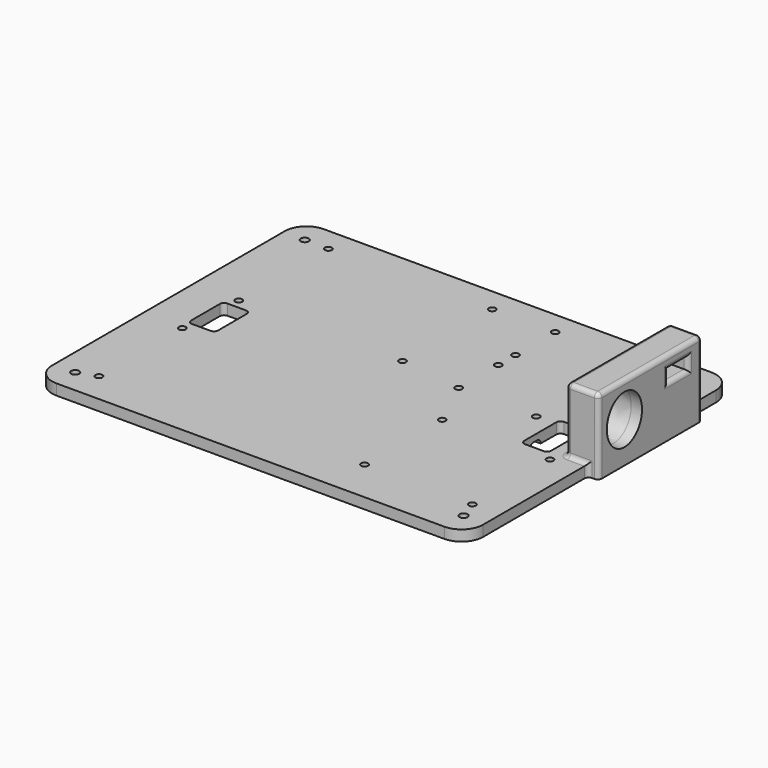
from build123d import *

# Parameters (mm, degrees)
F1_DEPTH  = 5
F2_R      = 1.85
F3_DEPTH  = 5
F2_R_2    = 2.595
F4_DEPTH  = 1.3
F5_DEPTH  = 2.17
F6_R      = 1.6
F7_DEPTH  = 3
F8_DEPTH  = 5
F9_W      = 12.5
F9_H      = 20.5508316867
F9_H_2    = 22.5
F10_DEPTH = 5
F9_W_2    = 10
F9_H_3    = 60
F9_W_3    = 5
F11_DEPTH = 30
F12_DEPTH = 5
F14_DEPTH = 10
F15_DEPTH = 5
F13_W     = 11.7
F13_H     = 5.3
F16_DEPTH = 10
F17_DEPTH = 5
F18_R     = 2
F19_R     = 2
F20_R     = 2


with BuildPart() as f1:
    # F0 (on Top) → F1 (new body)
    with BuildSketch(Plane.XY):
        with BuildLine():
            ThreePointArc((100, 67.5), (97.0710678119, 74.5710678119), (90, 77.5))
            Line((90, 77.5), (-90, 77.5))
            ThreePointArc((-90, 77.5), (-97.0710678119, 74.5710678119), (-100, 67.5))
            Line((-100, 67.5), (-100, -67.5))
            ThreePointArc((-100, -67.5), (-97.0710678119, -74.5710678119), (-90, -77.5))
            Line((-90, -77.5), (90, -77.5))
            ThreePointArc((90, -77.5), (97.0710678119, -74.5710678119), (100, -67.5))
            Line((100, -67.5), (100, 67.5))
        make_face()
    extrude(amount=F1_DEPTH)

    # F2 (on Top) → F3 (cut)
    with BuildSketch(Plane.XY):
        with Locations((-90.08, -66.5)):
            Circle(F2_R)
        with Locations((90.07, -66.42)):
            Circle(F2_R)
        with Locations((-90.05, 66.58)):
            Circle(F2_R)
        with Locations((89.94, 66.51)):
            Circle(F2_R)
    extrude(amount=F3_DEPTH, mode=Mode.SUBTRACT)

    # F2 (on Top) → F4 (cut)
    with BuildSketch(Plane.XY):
        with Locations((-62.465, -37.155)):
            Circle(F2_R_2)
        with Locations((-32.965, -37.295)):
            Circle(F2_R_2)
        with Locations((33.155, -36.905)):
            Circle(F2_R_2)
        with Locations((62.975, -37.145)):
            Circle(F2_R_2)
        with Locations((63.335, 37.005)):
            Circle(F2_R_2)
        with Locations((32.775, 37.335)):
            Circle(F2_R_2)
        with Locations((-33.385, 37.485)):
            Circle(F2_R_2)
        with Locations((-63.065, 37.835)):
            Circle(F2_R_2)
    extrude(amount=F4_DEPTH, mode=Mode.SUBTRACT)

    # F2 (on Top) → F5 (cut)
    with BuildSketch(Plane.XY):
        Polygon((-79.9484583735, -1.6147443093), (-79.9484583735, -3.4996026661), (-10.8238831162, -3.4996026661), (80.0515416265, -3.4996026661), (80.0515416265, 2.7003973339), (-79.9484583735, 2.7003973339), align=None)
    extrude(amount=F5_DEPTH, mode=Mode.SUBTRACT)

    # F6 (on Top) → F7 (cut)
    with BuildSketch(Plane.XY):
        Polygon((26, 37.2320508076), (23, 35.5), (23, 32.0358983849), (26, 30.3038475773), (29, 32.0358983849), (29, 35.5), align=None)
        with Locations((26, 33.7679491924)):
            Circle(F6_R, mode=Mode.SUBTRACT)
        Polygon((29, 42.0358983849), (29, 45.5), (26, 47.2320508076), (23, 45.5), (23, 42.0358983849), (26, 40.3038475773), align=None)
        with Locations((26, 43.7679491924)):
            Circle(F6_R, mode=Mode.SUBTRACT)
        Polygon((62, 47.2320508076), (59, 45.5), (59, 42.0358983849), (62, 40.3038475773), (65, 42.0358983849), (65, 45.5), align=None)
        with Locations((62, 43.7679491924)):
            Circle(F6_R, mode=Mode.SUBTRACT)
        Polygon((62, 37.2320508076), (59, 35.5), (59, 32.0358983849), (62, 30.3038475773), (65, 32.0358983849), (65, 35.5), align=None)
        with Locations((62, 33.7679491924)):
            Circle(F6_R, mode=Mode.SUBTRACT)
        Polygon((26, 70.2320508076), (23, 68.5), (23, 65.0358983849), (26, 63.3038475773), (29, 65.0358983849), (29, 68.5), align=None)
        with Locations((26, 66.7679491924)):
            Circle(F6_R, mode=Mode.SUBTRACT)
        Polygon((62, 70.2320508076), (59, 68.5), (59, 65.0358983849), (62, 63.3038475773), (65, 65.0358983849), (65, 68.5), align=None)
        with Locations((62, 66.7679491924)):
            Circle(F6_R, mode=Mode.SUBTRACT)
        Polygon((-3, 17.9641016151), (-6, 16.2320508076), (-6, 12.7679491924), (-3, 11.0358983849), (0, 12.7679491924), (0, 16.2320508076), align=None)
        with Locations((-3, 14.5)):
            Circle(F6_R, mode=Mode.SUBTRACT)
        Polygon((-76, 12.7679491924), (-76, 16.2320508076), (-79, 17.9641016151), (-82, 16.2320508076), (-82, 12.7679491924), (-79, 11.0358983849), align=None)
        with Locations((-79, 14.5)):
            Circle(F6_R, mode=Mode.SUBTRACT)
        Polygon((-79, 69.9641016151), (-82, 68.2320508076), (-82, 64.7679491924), (-79, 63.0358983849), (-76, 64.7679491924), (-76, 68.2320508076), align=None)
        with Locations((-79, 66.5)):
            Circle(F6_R, mode=Mode.SUBTRACT)
        Polygon((-81.386133541, -60.127273425), (-84.286133541, -61.8015892056), (-84.286133541, -65.1502207669), (-81.386133541, -66.8245365476), (-78.486133541, -65.1502207669), (-78.486133541, -61.8015892056), align=None)
        with Locations((-81.478695829, -63.4759049863)):
            Circle(F6_R, mode=Mode.SUBTRACT)
        Polygon((-81.478695829, -11.8017524848), (-84.378695829, -13.4760682655), (-84.378695829, -16.8246998268), (-81.478695829, -18.4990156074), (-78.578695829, -16.8246998268), (-78.578695829, -13.4760682655), align=None)
        with Locations((-81.478695829, -15.1503840461)):
            Circle(F6_R, mode=Mode.SUBTRACT)
        Polygon((87, -54.0358983849), (84, -55.7679491924), (84, -59.2320508076), (87, -60.9641016151), (90, -59.2320508076), (90, -55.7679491924), align=None)
        with Locations((87, -57.5)):
            Circle(F6_R, mode=Mode.SUBTRACT)
        Polygon((40, -59.2320508076), (40, -55.7679491924), (37, -54.0358983849), (34, -55.7679491924), (34, -59.2320508076), (37, -60.9641016151), align=None)
        with Locations((37, -57.5)):
            Circle(F6_R, mode=Mode.SUBTRACT)
        Polygon((37, -9.0358983849), (34, -10.7679491924), (34, -14.2320508076), (37, -15.9641016151), (40, -14.2320508076), (40, -10.7679491924), align=None)
        with Locations((37, -12.5)):
            Circle(F6_R, mode=Mode.SUBTRACT)
        Polygon((87, -9.0358983849), (84, -10.7679491924), (84, -14.2320508076), (87, -15.9641016151), (90, -14.2320508076), (90, -10.7679491924), align=None)
        with Locations((87, -12.5)):
            Circle(F6_R, mode=Mode.SUBTRACT)
        Polygon((29, 9.0358983849), (29, 12.5), (26, 14.2320508076), (23, 12.5), (23, 9.0358983849), (26, 7.3038475773), align=None)
        with Locations((26, 10.7679491924)):
            Circle(F6_R, mode=Mode.SUBTRACT)
        Polygon((-3, 69.9641016151), (-6, 68.2320508076), (-6, 64.7679491924), (-3, 63.0358983849), (0, 64.7679491924), (0, 68.2320508076), align=None)
        with Locations((-3, 66.5)):
            Circle(F6_R, mode=Mode.SUBTRACT)
        Polygon((62, 14.2320508076), (59, 12.5), (59, 9.0358983849), (62, 7.3038475773), (65, 9.0358983849), (65, 12.5), align=None)
        with Locations((62, 10.7679491924)):
            Circle(F6_R, mode=Mode.SUBTRACT)
    extrude(amount=F7_DEPTH, mode=Mode.SUBTRACT)

    # F6 (on Top) → F8 (cut)
    with BuildSketch(Plane.XY):
        with Locations((26, 10.7679491924)):
            Circle(F6_R)
        with Locations((37, -12.5)):
            Circle(F6_R)
        with Locations((26, 33.7679491924)):
            Circle(F6_R)
        with Locations((26, 43.7679491924)):
            Circle(F6_R)
        with Locations((26, 66.7679491924)):
            Circle(F6_R)
        with Locations((62, 66.7679491924)):
            Circle(F6_R)
        with Locations((62, 43.7679491924)):
            Circle(F6_R)
        with Locations((62, 33.7679491924)):
            Circle(F6_R)
        with Locations((87, -12.5)):
            Circle(F6_R)
        with Locations((87, -57.5)):
            Circle(F6_R)
        with Locations((37, -57.5)):
            Circle(F6_R)
        with Locations((-81.478695829, -63.4759049863)):
            Circle(F6_R)
        with Locations((-81.478695829, -15.1503840461)):
            Circle(F6_R)
        with Locations((-79, 14.5)):
            Circle(F6_R)
        with Locations((-3, 14.5)):
            Circle(F6_R)
        with Locations((-3, 66.5)):
            Circle(F6_R)
        with Locations((-79, 66.5)):
            Circle(F6_R)
        with Locations((62, 10.7679491924)):
            Circle(F6_R)
    extrude(amount=F8_DEPTH, mode=Mode.SUBTRACT)

    # F9 (on face) → F10 (cut)
    with BuildSketch(Plane.XY.offset(5)):
        with Locations((-76.45, -0.1583413687)):
            Rectangle(F9_W, F9_H)
        with Locations((76.75, 2.5285800407)):
            Rectangle(F9_W, F9_H_2)
    extrude(amount=-F10_DEPTH, mode=Mode.SUBTRACT)

    # F9 (on face) → F11 (join)
    with BuildSketch(Plane.XY.offset(5)):
        with Locations((95, 23.2044665329)):
            Rectangle(F9_W_2, F9_H_3)
        with Locations((102.5, 23.2044665329)):
            Rectangle(F9_W_3, F9_H_3)
    extrude(amount=F11_DEPTH)

    # F9 (on face) → F12 (join)
    with BuildSketch(Plane.XY.offset(5)):
        with Locations((102.5, 23.2044665329)):
            Rectangle(F9_W_3, F9_H_3)
    extrude(amount=-F12_DEPTH)

    # F13 (on face) → F14 (cut)
    with BuildSketch(Plane.YZ.offset(100)):
        with BuildLine():
            add(Edge.make_bspline(
                [(18.3977182999, 18.8161544502), (18.3977182999, 38.3883285757), (3.0977182999, 28.6022415129), (-12.2022817001, 18.8161544502), (3.0977182999, 9.0300673874), (18.3977182999, -0.7560196754), (18.3977182999, 18.8161544502)],
                knots=[4.7123889804, 4.7123889804, 4.7123889804, 6.8067840828, 6.8067840828, 8.9011791852, 8.9011791852, 10.9955742876, 10.9955742876, 10.9955742876], degree=2, weights=[1, 0.5, 1, 0.5, 1, 0.5, 1]))
        make_face()
    extrude(amount=-F14_DEPTH, mode=Mode.SUBTRACT)

    # F13 (on face) → F15 (cut)
    with BuildSketch(Plane.YZ.offset(100)):
        with BuildLine():
            add(Edge.make_bspline(
                [(18.3977182999, 18.8161544502), (18.3977182999, 38.3883285757), (3.0977182999, 28.6022415129), (-12.2022817001, 18.8161544502), (3.0977182999, 9.0300673874), (18.3977182999, -0.7560196754), (18.3977182999, 18.8161544502)],
                knots=[4.7123889804, 4.7123889804, 4.7123889804, 6.8067840828, 6.8067840828, 8.9011791852, 8.9011791852, 10.9955742876, 10.9955742876, 10.9955742876], degree=2, weights=[1, 0.5, 1, 0.5, 1, 0.5, 1]))
        make_face()
    extrude(amount=F15_DEPTH, mode=Mode.SUBTRACT)

    # F13 (on face) → F16 (cut)
    with BuildSketch(Plane.YZ.offset(100)):
        with Locations((39.3544665329, 26.35)):
            Rectangle(F13_W, F13_H)
    extrude(amount=-F16_DEPTH, mode=Mode.SUBTRACT)

    # F13 (on face) → F17 (cut)
    with BuildSketch(Plane.YZ.offset(100)):
        with Locations((39.3544665329, 26.35)):
            Rectangle(F13_W, F13_H)
    extrude(amount=F17_DEPTH, mode=Mode.SUBTRACT)

    # F18
    f18_edges = [f1.edges().sort_by_distance(p)[0] for p in [
        (0.15, -3.499603, 2.17),
        (0.15, 2.700397, 2.17),
    ]]
    fillet(f18_edges, radius=F18_R)

    # F19
    f19_edges = [f1.edges().sort_by_distance(p)[0] for p in [
        (97.5, -6.795533, 35),
        (97.5, 53.204467, 35),
        (105, -6.795533, 17.5),
        (105, 53.204467, 17.5),
        (90, 23.204467, 5),
        (95, -6.795533, 5),
        (95, 53.204467, 5),
        (100, 53.204467, 2.5),
        (100, -6.795533, 2.5),
        (90, 23.204467, 35),
        (90, 53.204467, 20),
        (90, -6.795533, 20),
        (105, 23.204467, 35),
        (105, 39.354467, 29),
        (105, 39.354467, 23.7),
        (105, 33.504467, 26.35),
        (105, 45.204467, 26.35),
        (90, 39.354467, 23.7),
        (90, 33.504467, 26.35),
        (90, 39.354467, 29),
        (90, 45.204467, 26.35),
    ]]
    fillet(f19_edges, radius=F19_R)

    # F20
    f20_edges = [f1.edges().sort_by_distance(p)[0] for p in [
        (-82.7, 10.117074, 2.5),
        (-70.2, 10.117074, 2.5),
        (-70.2, -10.433757, 2.5),
        (-82.7, -10.433757, 2.5),
        (83, -8.72142, 2.5),
        (70.5, -8.72142, 2.5),
        (83, 13.77858, 2.5),
        (70.5, 13.77858, 2.5),
    ]]
    fillet(f20_edges, radius=F20_R)


solid = f1.part
